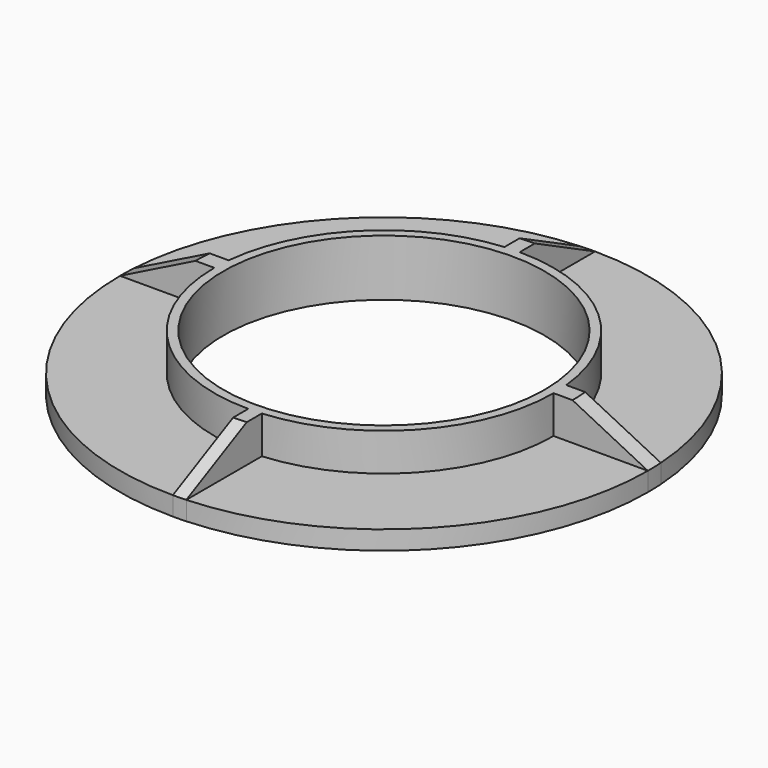
from build123d import *
from build123d import SkipClean  # not in build123d's __all__

# Parameters (mm, degrees)
F0_R        = 42.6
F1_DEPTH    = 5
F2_DEPTH    = 15
F3_DEPTH    = 3
F4_START    = 5
F4_DEPTH    = 10
F5_T2_ANGLE = 88.4610047723
F5_T4_ANGLE = 87.6524613708
F5_T6_ANGLE = 88.4610047722
F5_T8_ANGLE = 87.9917435352


# Not quite as in the source:
# - a fillet or chamfer that OpenCascade refuses, or shapes differently, is made with other operations: its cross-section is extruded or revolved along the edge and cut away or added


with BuildPart() as f1:
    # F0 (on Top) → F1 (new body)
    with BuildSketch(Plane.XY):
        with BuildLine():
            Line((45, 0), (70, 0))
            ThreePointArc((70, 0), (69.9641265525, 2.2407578514), (69.8565429786, 4.4792190254))
            Line((69.8565429786, 4.4792190254), (44.7765183654, 4.4792190254))
            ThreePointArc((44.7765183654, 4.4792190254), (44.9440948648, 2.2423953219), (45, 0))
        make_face()
        with BuildLine():
            Line((44.7765183654, 4.4792190254), (69.8565429786, 4.4792190254))
            ThreePointArc((69.8565429786, 4.4792190254), (47.8876532533, 51.0565633968), (0, 70))
            Line((0, 70), (0, 61.6992585301))
            ThreePointArc((0, 61.6992585301), (3.6415999231, 60.1908584533), (5.15, 56.5492585301))
            ThreePointArc((5.15, 56.5492585301), (3.6415999231, 52.907658607), (0, 51.3992585301))
            Line((0, 51.3992585301), (0, 45))
            ThreePointArc((0, 45), (30.194661315, 33.3658871914), (44.7765183654, 4.4792190254))
        make_face()
        with BuildLine():
            Line((0, 61.6992585301), (0, 70))
            ThreePointArc((0, 70), (-1.9542396645, 69.972715735), (-3.9069559007, 69.8908842095))
            Line((-3.9069559007, 69.8908842095), (-3.9069559007, 59.9045820004))
            ThreePointArc((-3.9069559007, 59.9045820004), (-2.1497190663, 61.2291311711), (0, 61.6992585301))
        make_face()
        with BuildLine():
            Line((-3.9069559007, 59.9045820004), (-3.9069559007, 69.8908842095))
            ThreePointArc((-3.9069559007, 69.8908842095), (-49.2943701377, 49.699749222), (-69.8565429786, 4.4792190254))
            Line((-69.8565429786, 4.4792190254), (-44.7765183654, 4.4792190254))
            ThreePointArc((-44.7765183654, 4.4792190254), (-31.6159465637, 32.0223659788), (-3.9069559007, 44.8300757928))
            Line((-3.9069559007, 44.8300757928), (-3.9069559007, 53.1939350599))
            ThreePointArc((-3.9069559007, 53.1939350599), (-5.15, 56.5492585301), (-3.9069559007, 59.9045820004))
        make_face()
        with BuildLine():
            ThreePointArc((-69.8565429786, 4.4792190254), (-69.9641265525, 2.2407578514), (-70, 0))
            Line((-70, 0), (-45, 0))
            ThreePointArc((-45, 0), (-44.9440948648, 2.2423953219), (-44.7765183654, 4.4792190254))
            Line((-44.7765183654, 4.4792190254), (-69.8565429786, 4.4792190254))
        make_face()
        with BuildLine():
            ThreePointArc((-70, 0), (-49.4974746831, -49.4974746831), (0, -70))
            Line((0, -70), (0, -45))
            ThreePointArc((0, -45), (-31.8198051534, -31.8198051534), (-45, 0))
            Line((-45, 0), (-70, 0))
        make_face()
        with BuildLine():
            ThreePointArc((0, -70), (1.7470617825, -69.9781949976), (3.4930351455, -69.9127935751))
            Line((3.4930351455, -69.9127935751), (3.4930351455, -44.8642252298))
            ThreePointArc((3.4930351455, -44.8642252298), (1.7478364709, -44.9660434959), (0, -45))
            Line((0, -45), (0, -70))
        make_face()
        with BuildLine():
            ThreePointArc((3.4930351455, -69.9127935751), (50.7174154516, -48.2466969844), (70, 0))
            Line((70, 0), (45, 0))
            ThreePointArc((45, 0), (33.0317013, -30.5598872581), (3.4930351455, -44.8642252298))
            Line((3.4930351455, -44.8642252298), (3.4930351455, -69.9127935751))
        make_face()
        with BuildLine():
            Line((0, 51.3992585301), (0, 61.6992585301))
            ThreePointArc((0, 61.6992585301), (-2.1497190663, 61.2291311711), (-3.9069559007, 59.9045820004))
            Line((-3.9069559007, 59.9045820004), (-3.9069559007, 53.1939350599))
            ThreePointArc((-3.9069559007, 53.1939350599), (-2.1497190663, 51.8693858891), (0, 51.3992585301))
        make_face()
        with BuildLine():
            Line((-3.9069559007, 53.1939350599), (-3.9069559007, 59.9045820004))
            ThreePointArc((-3.9069559007, 59.9045820004), (-5.15, 56.5492585301), (-3.9069559007, 53.1939350599))
        make_face()
        with BuildLine():
            ThreePointArc((5.15, 56.5492585301), (3.6415999231, 60.1908584533), (0, 61.6992585301))
            Line((0, 61.6992585301), (0, 51.3992585301))
            ThreePointArc((0, 51.3992585301), (3.6415999231, 52.907658607), (5.15, 56.5492585301))
        make_face()
        with BuildLine():
            ThreePointArc((-3.9069559007, 44.8300757928), (-1.9553246946, 44.9574988777), (0, 45))
            Line((0, 45), (0, 51.3992585301))
            ThreePointArc((0, 51.3992585301), (-2.1497190663, 51.8693858891), (-3.9069559007, 53.1939350599))
            Line((-3.9069559007, 53.1939350599), (-3.9069559007, 44.8300757928))
        make_face()
        with BuildLine():
            ThreePointArc((3.4930351455, -44.8642252298), (33.0317013, -30.5598872581), (45, 0))
            ThreePointArc((45, 0), (44.9440948648, 2.2423953219), (44.7765183654, 4.4792190254))
            ThreePointArc((44.7765183654, 4.4792190254), (30.194661315, 33.3658871914), (0, 45))
            ThreePointArc((0, 45), (-1.9553246946, 44.9574988777), (-3.9069559007, 44.8300757928))
            ThreePointArc((-3.9069559007, 44.8300757928), (-31.6159465637, 32.0223659788), (-44.7765183654, 4.4792190254))
            ThreePointArc((-44.7765183654, 4.4792190254), (-44.9440948648, 2.2423953219), (-45, 0))
            ThreePointArc((-45, 0), (-31.8198051534, -31.8198051534), (0, -45))
            ThreePointArc((0, -45), (1.7478364709, -44.9660434959), (3.4930351455, -44.8642252298))
        make_face()
        Circle(F0_R, mode=Mode.SUBTRACT)
    extrude(amount=F1_DEPTH)

    # F0 (on Top) → F2 (join)
    with BuildSketch(Plane.XY):
        with BuildLine():
            ThreePointArc((3.4930351455, -44.8642252298), (33.0317013, -30.5598872581), (45, 0))
            ThreePointArc((45, 0), (44.9440948648, 2.2423953219), (44.7765183654, 4.4792190254))
            ThreePointArc((44.7765183654, 4.4792190254), (30.194661315, 33.3658871914), (0, 45))
            ThreePointArc((0, 45), (-1.9553246946, 44.9574988777), (-3.9069559007, 44.8300757928))
            ThreePointArc((-3.9069559007, 44.8300757928), (-31.6159465637, 32.0223659788), (-44.7765183654, 4.4792190254))
            ThreePointArc((-44.7765183654, 4.4792190254), (-44.9440948648, 2.2423953219), (-45, 0))
            ThreePointArc((-45, 0), (-31.8198051534, -31.8198051534), (0, -45))
            ThreePointArc((0, -45), (1.7478364709, -44.9660434959), (3.4930351455, -44.8642252298))
        make_face()
        Circle(F0_R, mode=Mode.SUBTRACT)
    extrude(amount=F2_DEPTH)

    # F0 (on Top) → F3 (cut)
    with BuildSketch(Plane.XY):
        with BuildLine():
            Line((0, 51.3992585301), (0, 61.6992585301))
            ThreePointArc((0, 61.6992585301), (-2.1497190663, 61.2291311711), (-3.9069559007, 59.9045820004))
            Line((-3.9069559007, 59.9045820004), (-3.9069559007, 53.1939350599))
            ThreePointArc((-3.9069559007, 53.1939350599), (-2.1497190663, 51.8693858891), (0, 51.3992585301))
        make_face()
        with BuildLine():
            ThreePointArc((5.15, 56.5492585301), (3.6415999231, 60.1908584533), (0, 61.6992585301))
            Line((0, 61.6992585301), (0, 51.3992585301))
            ThreePointArc((0, 51.3992585301), (3.6415999231, 52.907658607), (5.15, 56.5492585301))
        make_face()
        with BuildLine():
            Line((-3.9069559007, 53.1939350599), (-3.9069559007, 59.9045820004))
            ThreePointArc((-3.9069559007, 59.9045820004), (-5.15, 56.5492585301), (-3.9069559007, 53.1939350599))
        make_face()
    extrude(amount=F3_DEPTH, mode=Mode.SUBTRACT)

    # F0 (on Top) → F4 (join)
    with BuildSketch(Plane.XY.offset(F4_START)):
        with BuildLine():
            ThreePointArc((0, -70), (1.7470617825, -69.9781949976), (3.4930351455, -69.9127935751))
            Line((3.4930351455, -69.9127935751), (3.4930351455, -44.8642252298))
            ThreePointArc((3.4930351455, -44.8642252298), (1.7478364709, -44.9660434959), (0, -45))
            Line((0, -45), (0, -70))
        make_face()
        with BuildLine():
            ThreePointArc((-69.8565429786, 4.4792190254), (-69.9641265525, 2.2407578514), (-70, 0))
            Line((-70, 0), (-45, 0))
            ThreePointArc((-45, 0), (-44.9440948648, 2.2423953219), (-44.7765183654, 4.4792190254))
            Line((-44.7765183654, 4.4792190254), (-69.8565429786, 4.4792190254))
        make_face()
        with BuildLine():
            Line((45, 0), (70, 0))
            ThreePointArc((70, 0), (69.9641265525, 2.2407578514), (69.8565429786, 4.4792190254))
            Line((69.8565429786, 4.4792190254), (44.7765183654, 4.4792190254))
            ThreePointArc((44.7765183654, 4.4792190254), (44.9440948648, 2.2423953219), (45, 0))
        make_face()
        with BuildLine():
            Line((0, 51.3992585301), (0, 61.6992585301))
            ThreePointArc((0, 61.6992585301), (-2.1497190663, 61.2291311711), (-3.9069559007, 59.9045820004))
            Line((-3.9069559007, 59.9045820004), (-3.9069559007, 53.1939350599))
            ThreePointArc((-3.9069559007, 53.1939350599), (-2.1497190663, 51.8693858891), (0, 51.3992585301))
        make_face()
        with BuildLine():
            Line((0, 61.6992585301), (0, 70))
            ThreePointArc((0, 70), (-1.9542396645, 69.972715735), (-3.9069559007, 69.8908842095))
            Line((-3.9069559007, 69.8908842095), (-3.9069559007, 59.9045820004))
            ThreePointArc((-3.9069559007, 59.9045820004), (-2.1497190663, 61.2291311711), (0, 61.6992585301))
        make_face()
        with BuildLine():
            ThreePointArc((-3.9069559007, 44.8300757928), (-1.9553246946, 44.9574988777), (0, 45))
            Line((0, 45), (0, 51.3992585301))
            ThreePointArc((0, 51.3992585301), (-2.1497190663, 51.8693858891), (-3.9069559007, 53.1939350599))
            Line((-3.9069559007, 53.1939350599), (-3.9069559007, 44.8300757928))
        make_face()
    with SkipClean():  # cleaning this boolean's faces spoils the solid; the shape is the same uncleaned
        extrude(amount=F4_DEPTH)

    # F5: chamfer of 20 x 10 on 4 edges, made by hand

    # F5_s1 → F5_t2 (revolve, cut)
    with BuildSketch(Plane(origin=(0, 0, 0), x_dir=(0, 0, 1), z_dir=(-0.6742521694, -0.738501193, 0))):
        Polygon((5, -70), (15, -50), (15, -70), align=None)
    revolve(axis=Axis((0, 0, 15), (0, 0, 1)), revolution_arc=F5_T2_ANGLE, mode=Mode.SUBTRACT)

    # F5_s3 → F5_t4 (revolve, cut)
    with BuildSketch(Plane(origin=(0, 0, 0), x_dir=(0, 0, 1), z_dir=(-0.7385013236, 0.6742520264, 0))):
        Polygon((5, -70), (15, -50), (15, -70), align=None)
    revolve(axis=Axis((0, 0, 15), (0, 0, 1)), revolution_arc=F5_T4_ANGLE, mode=Mode.SUBTRACT)

    # F5_s5 → F5_t6 (revolve, cut)
    with BuildSketch(Plane(origin=(0, 0, 0), x_dir=(0, 0, 1), z_dir=(0.7201262035, 0.6938431026, 0))):
        Polygon((5, -70), (15, -50), (15, -70), align=None)
    revolve(axis=Axis((0, 0, 15), (0, 0, 1)), revolution_arc=F5_T6_ANGLE, mode=Mode.SUBTRACT)

    # F5_s7 → F5_t8 (revolve, cut)
    with BuildSketch(Plane(origin=(0, 0, 0), x_dir=(0, 0, 1), z_dir=(0.7385012727, -0.6742520821, 0))):
        Polygon((5, -70), (15, -50), (15, -70), align=None)
    revolve(axis=Axis((0, 0, 15), (0, 0, 1)), revolution_arc=F5_T8_ANGLE, mode=Mode.SUBTRACT)


solid = f1.part
